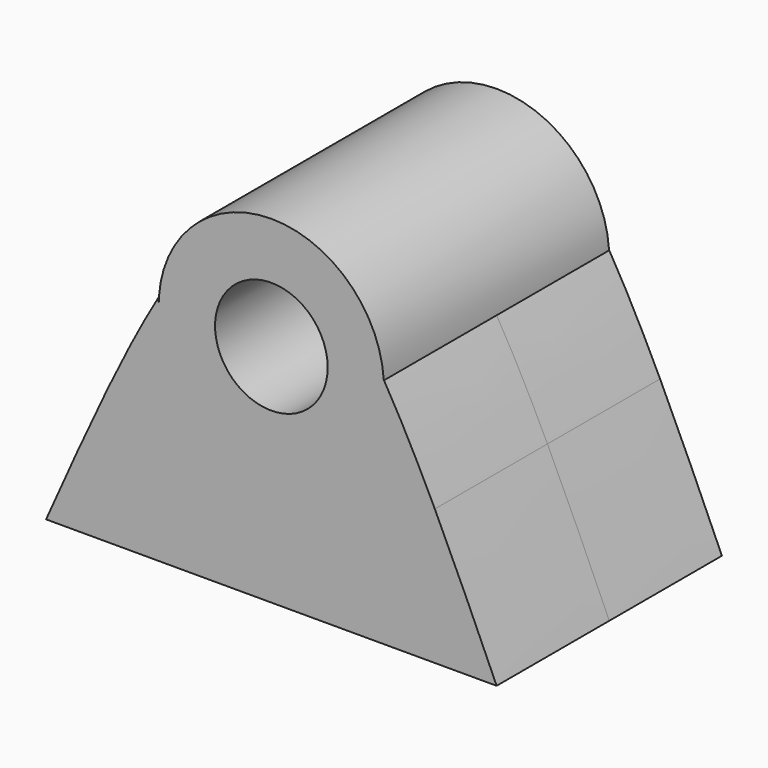
from build123d import *

# Parameters (mm, degrees)
F2_DEPTH = 12.5
F0_R     = 5
F3_DEPTH = 12.5


with BuildPart() as f2:
    # F1 (on Front) → F2 (new body, symmetric)
    with BuildSketch(Plane.XZ):
        with BuildLine():
            Line((-10, 0), (10, 0))
            Line((10, 0), (10, 12.0382448658))
            Line((10, 12.0382448658), (6.0506574175, 12.0382448658))
            ThreePointArc((6.0506574175, 12.0382448658), (0, 10), (-6.0506574175, 12.0382448658))
            Line((-6.0506574175, 12.0382448658), (-10, 12.0382448658))
            Line((-10, 12.0382448658), (-10, 0))
        make_face()
        with BuildLine():
            Line((10, 12.0382448658), (10, 0))
            Line((10, 0), (20, 0))
            add(Edge.make_bspline(
                [(14.5119228257, 12.0382448658), (16.3412818838, 8.2321157615), (18.1706409419, 4.1160578807), (20, 0)],
                knots=[0.8627980706, 0.8627980706, 0.8627980706, 0.8627980706, 1, 1, 1, 1], degree=3))
            Line((14.5119228257, 12.0382448658), (10, 12.0382448658))
        make_face()
        with BuildLine():
            Line((-20, 0), (-10, 0))
            Line((-10, 0), (-10, 12.0382448658))
            Line((-10, 12.0382448658), (-14.5119228257, 12.0382448658))
            add(Edge.make_bspline(
                [(-20, 0), (-18.1706409419, 4.1160578807), (-16.3412818838, 8.2321157615), (-14.5119228257, 12.0382448658)],
                knots=[0, 0, 0, 0, 0.1372019294, 0.1372019294, 0.1372019294, 0.1372019294], degree=3))
        make_face()
        with BuildLine():
            Line((6.0506574175, 12.0382448658), (10, 12.0382448658))
            Line((10, 12.0382448658), (10, 20))
            ThreePointArc((10, 20), (8.958419899, 15.556272633), (6.0506574175, 12.0382448658))
        make_face()
        with BuildLine():
            Line((10, 20), (10, 12.0382448658))
            Line((10, 12.0382448658), (14.5119228257, 12.0382448658))
            add(Edge.make_bspline(
                [(10, 20.625), (11.5039742752, 18.0870434106), (13.0079485504, 15.1673846789), (14.5119228257, 12.0382448658)],
                knots=[0.75, 0.75, 0.75, 0.75, 0.8627980706, 0.8627980706, 0.8627980706, 0.8627980706], degree=3))
            Line((10, 20.625), (10, 20))
        make_face()
        with BuildLine():
            Line((-14.5119228257, 12.0382448658), (-10, 12.0382448658))
            Line((-10, 12.0382448658), (-10, 20))
            Line((-10, 20), (-10, 20.625))
            add(Edge.make_bspline(
                [(-14.5119228257, 12.0382448658), (-13.0079485504, 15.1673846789), (-11.5039742752, 18.0870434106), (-10, 20.625)],
                knots=[0.1372019294, 0.1372019294, 0.1372019294, 0.1372019294, 0.25, 0.25, 0.25, 0.25], degree=3))
        make_face()
        with BuildLine():
            Line((-10, 20), (-10, 12.0382448658))
            Line((-10, 12.0382448658), (-6.0506574175, 12.0382448658))
            ThreePointArc((-6.0506574175, 12.0382448658), (-8.958419899, 15.556272633), (-10, 20))
        make_face()
        with BuildLine():
            ThreePointArc((6.0506574175, 12.0382448658), (8.958419899, 15.556272633), (10, 20))
            ThreePointArc((10, 20), (9.9945146107, 20.3311762316), (9.9780644607, 20.661989137))
            add(Edge.make_bspline(
                [(0, 30), (3.3260214869, 30), (6.6520429738, 26.2664336107), (9.9780644607, 20.661989137)],
                knots=[0.5, 0.5, 0.5, 0.5, 0.7494516115, 0.7494516115, 0.7494516115, 0.7494516115], degree=3))
            add(Edge.make_bspline(
                [(-9.9780644607, 20.661989137), (-6.6520429738, 26.2664336107), (-3.3260214869, 30), (0, 30)],
                knots=[0.2505483885, 0.2505483885, 0.2505483885, 0.2505483885, 0.5, 0.5, 0.5, 0.5], degree=3))
            ThreePointArc((-9.9780644607, 20.661989137), (-9.9945146107, 20.3311762316), (-10, 20))
            ThreePointArc((-10, 20), (-8.958419899, 15.556272633), (-6.0506574175, 12.0382448658))
            Line((-6.0506574175, 12.0382448658), (6.0506574175, 12.0382448658))
        make_face()
        with BuildLine():
            ThreePointArc((-6.0506574175, 12.0382448658), (0, 10), (6.0506574175, 12.0382448658))
            Line((6.0506574175, 12.0382448658), (-6.0506574175, 12.0382448658))
        make_face()
        with BuildLine():
            add(Edge.make_bspline(
                [(0, 30), (3.3260214869, 30), (6.6520429738, 26.2664336107), (9.9780644607, 20.661989137)],
                knots=[0.5, 0.5, 0.5, 0.5, 0.7494516115, 0.7494516115, 0.7494516115, 0.7494516115], degree=3))
            ThreePointArc((9.9780644607, 20.661989137), (6.8330120968, 27.301366015), (0, 30))
        make_face()
        with BuildLine():
            ThreePointArc((0, 30), (-6.8330120968, 27.301366015), (-9.9780644607, 20.661989137))
            add(Edge.make_bspline(
                [(-9.9780644607, 20.661989137), (-6.6520429738, 26.2664336107), (-3.3260214869, 30), (0, 30)],
                knots=[0.2505483885, 0.2505483885, 0.2505483885, 0.2505483885, 0.5, 0.5, 0.5, 0.5], degree=3))
        make_face()
    extrude(amount=F2_DEPTH, both=True)

    # F0 (on Front) → F3 (cut, symmetric)
    with BuildSketch(Plane.XZ):
        with Locations((0, 20)):
            Circle(F0_R)
    extrude(amount=F3_DEPTH, both=True, mode=Mode.SUBTRACT)


solid = f2.part
